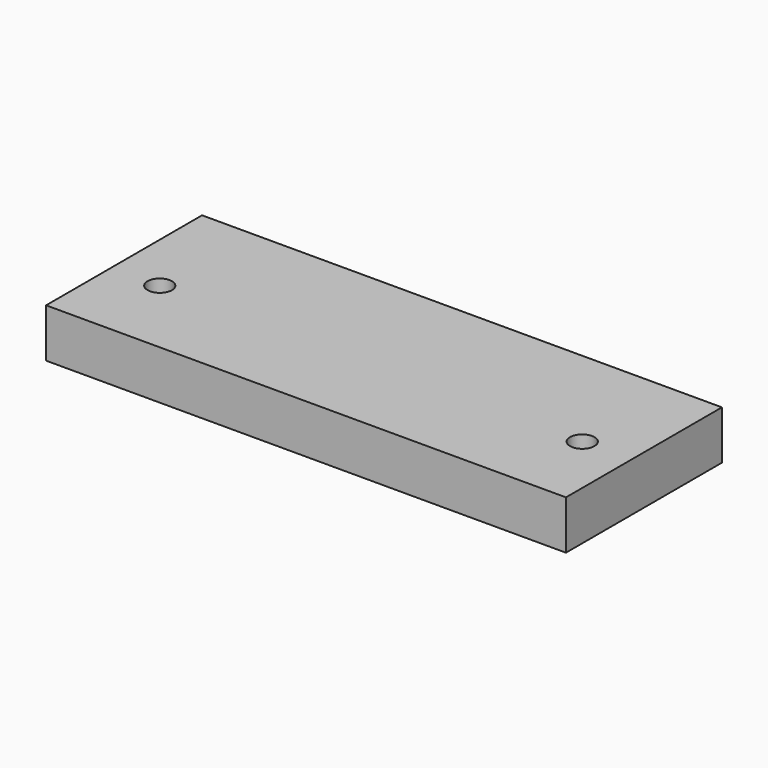
from build123d import *

# Parameters (mm, degrees)
F0_W     = 50.8
F0_H     = 19.05
F3_DEPTH = 4.7625
F2_R     = 1.1938
F4_DEPTH = 4.7625
F1_R     = 1.190625
F5_DEPTH = 4.7625


# Not quite as in the source:
# - a length typed as a fraction of an inch, garbled in the dataset ("3 / 203.2 mm" for 3/8 in), is restored


with BuildPart() as f3:
    # F0 (on Top) → F3 (new body)
    with BuildSketch(Plane.XY):
        Rectangle(F0_W, F0_H)
    extrude(amount=F3_DEPTH)

    # F2 (on face) → F4 (cut)
    with BuildSketch(Plane.XY):
        with Locations((20.6155478954, -1.5542221954)):
            Circle(F2_R)
    extrude(amount=F4_DEPTH, mode=Mode.SUBTRACT)

    # F1 (on face) → F5 (cut)
    with BuildSketch(Plane.XY):
        with Locations((-20.6543747336, -1.571108005)):
            Circle(F1_R)
    extrude(amount=F5_DEPTH, mode=Mode.SUBTRACT)


solid = f3.part
